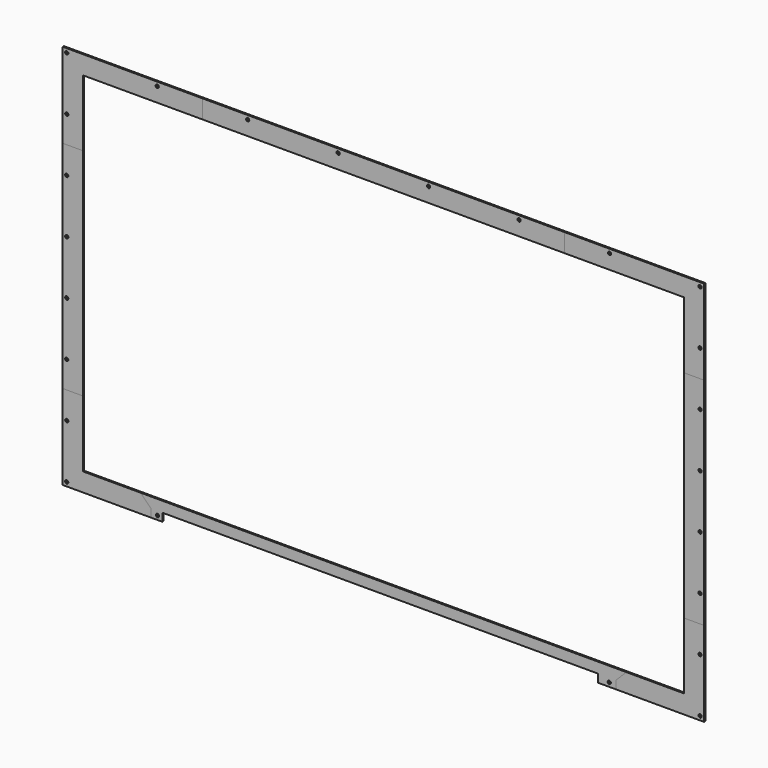
from build123d import *

# Parameters (mm, degrees)
F0_R     = 2.54
F1_DEPTH = 1.1811
F0_W     = 573.314286
F0_H     = 16.66875
F2_DEPTH = 1.1811
F3_DEPTH = 1.1811
F0_W_2   = 19.304
F0_H_2   = 341.992858
F0_W_3   = 12.7
F4_DEPTH = 1.1811
F5_DEPTH = 1.1811
F0_W_4   = 28.00096
F0_H_3   = 12.7
F0_W_5   = 18.00098
F6_DEPTH = 1.1811
F7_DEPTH = 1.1811
F8_DEPTH = 1.1811


# Not quite as in the source:
# - a feature names something its author has since deleted; it is built from what else it names


with BuildPart() as f1:
    # F0 (on Front) → F1 (new body, symmetric)
    with BuildSketch(Plane.XZ):
        Polygon((-286.657143, 276.225), (-286.657143, 292.89375), (-495.3, 292.89375), (-495.3, 170.996429), (-475.996, 170.996429), (-475.996, 276.225), align=None)
        with BuildLine():
            Line((-495.3, 170.996429), (-495.3, 292.89375))
            Line((-495.3, 292.89375), (-499.853949, 297.447699))
            ThreePointArc((-499.853949, 297.447699), (-503.446051, 297.447699), (-503.446051, 301.039801))
            Line((-503.446051, 301.039801), (-508, 305.59375))
            Line((-508, 305.59375), (-508, 170.996429))
            Line((-508, 170.996429), (-501.65, 170.996429))
            Line((-501.65, 170.996429), (-495.3, 170.996429))
        make_face()
        with BuildLine():
            ThreePointArc((-499.11, 213.745536), (-499.853949, 211.949484), (-501.65, 211.205536))
            ThreePointArc((-501.65, 211.205536), (-503.446051, 215.541587), (-499.11, 213.745536))
        make_face(mode=Mode.SUBTRACT)
        with BuildLine():
            Line((-495.3, 292.89375), (-286.657143, 292.89375))
            Line((-286.657143, 292.89375), (-286.657143, 299.24375))
            Line((-286.657143, 299.24375), (-286.657143, 305.59375))
            Line((-286.657143, 305.59375), (-508, 305.59375))
            Line((-508, 305.59375), (-503.446051, 301.039801))
            ThreePointArc((-503.446051, 301.039801), (-500.677984, 301.590404), (-499.11, 299.24375))
            ThreePointArc((-499.11, 299.24375), (-499.303346, 298.271734), (-499.853949, 297.447699))
            Line((-499.853949, 297.447699), (-495.3, 292.89375))
        make_face()
        with Locations((-358.321429, 299.24375)):
            Circle(F0_R, mode=Mode.SUBTRACT)
    extrude(amount=F1_DEPTH, both=True)


with BuildPart() as f2:
    # F0 (on Front) → F2 (new body, symmetric)
    with BuildSketch(Plane.XZ):
        with Locations((0, 284.559375)):
            Rectangle(F0_W, F0_H)
        Polygon((-286.657143, 292.89375), (286.657143, 292.89375), (286.657143, 305.59375), (-286.657143, 305.59375), (-286.657143, 299.24375), align=None)
        with BuildLine():
            ThreePointArc((-212.452857, 299.24375), (-214.992857, 296.70375), (-217.532857, 299.24375))
            ThreePointArc((-217.532857, 299.24375), (-214.992857, 301.78375), (-212.452857, 299.24375))
        make_face(mode=Mode.SUBTRACT)
        with Locations((-71.664286, 299.24375)):
            Circle(F0_R, mode=Mode.SUBTRACT)
        with Locations((71.664286, 299.24375)):
            Circle(F0_R, mode=Mode.SUBTRACT)
        with Locations((214.992857, 299.24375)):
            Circle(F0_R, mode=Mode.SUBTRACT)
    extrude(amount=F2_DEPTH, both=True)


with BuildPart() as f3:
    # F0 (on Front) → F3 (new body, symmetric)
    with BuildSketch(Plane.XZ):
        Polygon((495.3, 170.996429), (495.3, 292.89375), (286.657143, 292.89375), (286.657143, 276.225), (475.996, 276.225), (475.996, 170.996429), align=None)
        Polygon((286.657143, 292.89375), (495.3, 292.89375), (495.3, 170.996429), (508, 170.996429), (508, 305.59375), (286.657143, 305.59375), align=None)
        with Locations((501.65, 213.745536)):
            Circle(F0_R, mode=Mode.SUBTRACT)
        with Locations((358.321429, 299.24375)):
            Circle(F0_R, mode=Mode.SUBTRACT)
        with Locations((501.65, 299.24375)):
            Circle(F0_R, mode=Mode.SUBTRACT)
    extrude(amount=F3_DEPTH, both=True)


with BuildPart() as f4:
    # F0 (on Front) → F4 (new body, symmetric)
    with BuildSketch(Plane.XZ):
        with Locations((485.648, 0)):
            Rectangle(F0_W_2, F0_H_2)
        with Locations((501.65, 0)):
            Rectangle(F0_W_3, F0_H_2)
        with Locations((501.65, -128.247321)):
            Circle(F0_R, mode=Mode.SUBTRACT)
        with Locations((501.65, -42.749107)):
            Circle(F0_R, mode=Mode.SUBTRACT)
        with Locations((501.65, 42.749107)):
            Circle(F0_R, mode=Mode.SUBTRACT)
        with Locations((501.65, 128.247321)):
            Circle(F0_R, mode=Mode.SUBTRACT)
    extrude(amount=F4_DEPTH, both=True)


with BuildPart() as f5:
    # F0 (on Front) → F5 (new body, symmetric)
    with BuildSketch(Plane.XZ):
        Polygon((508, -170.996429), (495.3, -170.996429), (495.3, -292.89375), (368.3, -292.89375), (368.3, -305.59375), (508, -305.59375), align=None)
        with Locations((501.65, -299.24375)):
            Circle(F0_R, mode=Mode.SUBTRACT)
        with Locations((501.65, -213.745536)):
            Circle(F0_R, mode=Mode.SUBTRACT)
        Polygon((495.3, -292.89375), (495.3, -170.996429), (475.996, -170.996429), (475.996, -276.225), (384.96875, -276.225), (368.3, -292.89375), align=None)
    extrude(amount=F5_DEPTH, both=True)


with BuildPart() as f6:
    # F0 (on Front) → F6 (new body, symmetric)
    with BuildSketch(Plane.XZ):
        Polygon((340.29904, -292.89375), (368.3, -292.89375), (384.96875, -276.225), (-384.96875, -276.225), (-368.3, -292.89375), (-350.29902, -292.89375), align=None)
        with Locations((354.29952, -299.24375)):
            Rectangle(F0_W_4, F0_H_3)
        with Locations((357.84, -299.24375)):
            Circle(F0_R, mode=Mode.SUBTRACT)
        with Locations((-359.29951, -299.24375)):
            Rectangle(F0_W_5, F0_H_3)
        with Locations((-357.84, -299.24375)):
            Circle(F0_R, mode=Mode.SUBTRACT)
    extrude(amount=F6_DEPTH, both=True)


with BuildPart() as f7:
    # F0 (on Front) → F7 (new body, symmetric)
    with BuildSketch(Plane.XZ):
        with BuildLine():
            Line((-368.3, -292.89375), (-495.3, -292.89375))
            Line((-495.3, -292.89375), (-499.853949, -297.447699))
            ThreePointArc((-499.853949, -297.447699), (-499.303346, -298.271734), (-499.11, -299.24375))
            ThreePointArc((-499.11, -299.24375), (-500.677984, -301.590404), (-503.446051, -301.039801))
            Line((-503.446051, -301.039801), (-508, -305.59375))
            Line((-508, -305.59375), (-368.3, -305.59375))
            Line((-368.3, -305.59375), (-368.3, -292.89375))
        make_face()
        with BuildLine():
            Line((-495.3, -292.89375), (-495.3, -170.996429))
            Line((-495.3, -170.996429), (-508, -170.996429))
            Line((-508, -170.996429), (-508, -305.59375))
            Line((-508, -305.59375), (-503.446051, -301.039801))
            ThreePointArc((-503.446051, -301.039801), (-503.446051, -297.447699), (-499.853949, -297.447699))
            Line((-499.853949, -297.447699), (-495.3, -292.89375))
        make_face()
        with Locations((-501.65, -213.745536)):
            Circle(F0_R, mode=Mode.SUBTRACT)
        Polygon((-475.996, -170.996429), (-495.3, -170.996429), (-495.3, -292.89375), (-368.3, -292.89375), (-384.96875, -276.225), (-475.996, -276.225), align=None)
    extrude(amount=F7_DEPTH, both=True)


with BuildPart() as f8:
    # F0 (on Front) → F8 (new body, symmetric)
    with BuildSketch(Plane.XZ):
        with Locations((-485.648, 0)):
            Rectangle(F0_W_2, F0_H_2)
        Polygon((-495.3, -170.996429), (-495.3, 170.996429), (-501.65, 170.996429), (-508, 170.996429), (-508, -170.996429), align=None)
        with Locations((-501.65, -128.247321)):
            Circle(F0_R, mode=Mode.SUBTRACT)
        with Locations((-501.65, -42.749107)):
            Circle(F0_R, mode=Mode.SUBTRACT)
        with Locations((-501.65, 42.749107)):
            Circle(F0_R, mode=Mode.SUBTRACT)
        with BuildLine():
            ThreePointArc((-499.11, 128.247321), (-503.446051, 126.45127), (-501.65, 130.787321))
            ThreePointArc((-501.65, 130.787321), (-499.853949, 130.043373), (-499.11, 128.247321))
        make_face(mode=Mode.SUBTRACT)
    extrude(amount=F8_DEPTH, both=True)


solid = Compound([f1.part, f2.part, f3.part, f4.part, f5.part, f6.part, f7.part, f8.part])
